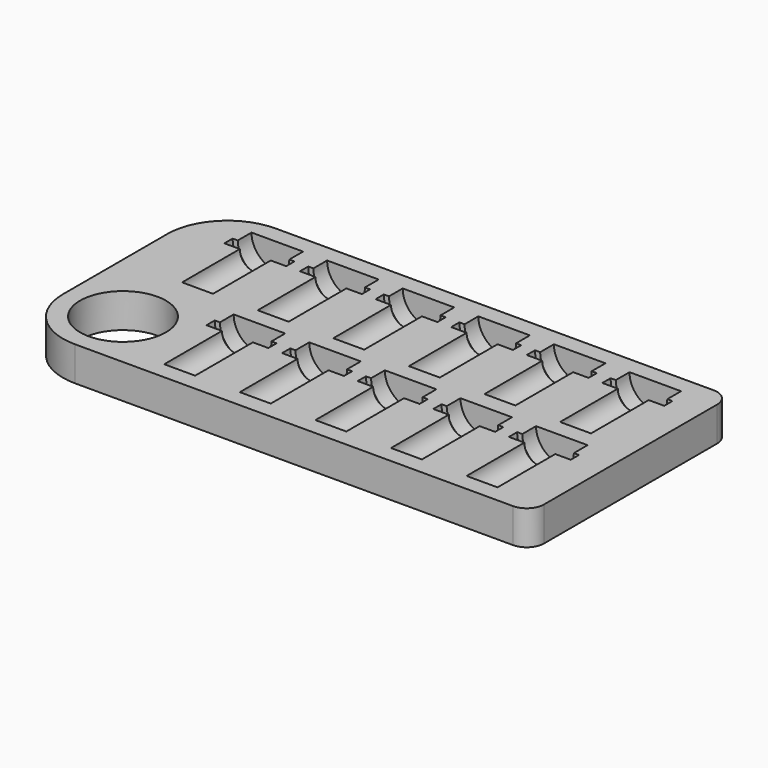
from build123d import *

# Parameters (mm, degrees)
F0_R         = 12.5
F1_DEPTH     = 10
F9_TEXT_SIZE = 5.5555555556
F10_DEPTH    = 1


# Not quite as in the source:
# - Text() gives the source's letters only with a copy of the font that has no kerning and outlines rounded to 1/6400 em; it was checked with that copy


with BuildPart() as f1:
    # F0 (on Top) → F1 (new body)
    with BuildSketch(Plane.XY):
        with BuildLine():
            ThreePointArc((0, 17.5), (5.1256313292, 5.1256313292), (17.5, 0))
            Line((17.5, 0), (145, 0))
            ThreePointArc((145, 0), (148.5355339059, 1.4644660941), (150, 5))
            Line((150, 5), (150, 68))
            ThreePointArc((150, 68), (148.5355339059, 71.5355339059), (145, 73))
            Line((145, 73), (17.5, 73))
            ThreePointArc((17.5, 73), (5.1256313292, 67.8743686708), (0, 55.5))
            Line((0, 55.5), (0, 17.5))
        make_face()
        with Locations((17.5, 17.5)):
            Circle(F0_R, mode=Mode.SUBTRACT)
    extrude(amount=F1_DEPTH)

    # F2 (on face) → F3 (revolve, cut)
    with BuildSketch(Plane.XY.offset(10)):
        Polygon((22, 60), (22, 39), (26.5, 39), (26.5, 60), (31, 60), (31, 63), (29.5, 63), (29.5, 68), (22, 68), (22, 63), align=None)
    revolve(axis=Axis((22, 49.5, 10), (0, 1, 0)), mode=Mode.SUBTRACT)

    # F2 (on face) → F4 (revolve, cut)
    with BuildSketch(Plane.XY.offset(10)):
        Polygon((44, 26), (44, 5), (48.5, 5), (48.5, 26), (53, 26), (53, 29), (51.5, 29), (51.5, 34), (44, 34), (44, 29), align=None)
        Polygon((44, 60), (44, 39), (48.5, 39), (48.5, 60), (53, 60), (53, 63), (51.5, 63), (51.5, 68), (44, 68), (44, 63), align=None)
    revolve(axis=Axis((44, 49.5, 10), (0, 1, 0)), mode=Mode.SUBTRACT)

    # F2 (on face) → F5 (revolve, cut)
    with BuildSketch(Plane.XY.offset(10)):
        Polygon((66, 26), (66, 5), (70.5, 5), (70.5, 26), (75, 26), (75, 29), (73.5, 29), (73.5, 34), (66, 34), (66, 29), align=None)
        Polygon((66, 60), (66, 39), (70.5, 39), (70.5, 60), (75, 60), (75, 63), (73.5, 63), (73.5, 68), (66, 68), (66, 63), align=None)
    revolve(axis=Axis((66, 49.5, 10), (0, 1, 0)), mode=Mode.SUBTRACT)

    # F2 (on face) → F6 (revolve, cut)
    with BuildSketch(Plane.XY.offset(10)):
        Polygon((88, 26), (88, 5), (92.5, 5), (92.5, 26), (97, 26), (97, 29), (95.5, 29), (95.5, 34), (88, 34), (88, 29), align=None)
        Polygon((88, 60), (88, 39), (92.5, 39), (92.5, 60), (97, 60), (97, 63), (95.5, 63), (95.5, 68), (88, 68), (88, 63), align=None)
    revolve(axis=Axis((88, 49.5, 10), (0, 1, 0)), mode=Mode.SUBTRACT)

    # F2 (on face) → F7 (revolve, cut)
    with BuildSketch(Plane.XY.offset(10)):
        Polygon((110, 26), (110, 5), (114.5, 5), (114.5, 26), (119, 26), (119, 29), (117.5, 29), (117.5, 34), (110, 34), (110, 29), align=None)
        Polygon((110, 60), (110, 39), (114.5, 39), (114.5, 60), (119, 60), (119, 63), (117.5, 63), (117.5, 68), (110, 68), (110, 63), align=None)
    revolve(axis=Axis((110, 49.5, 10), (0, 1, 0)), mode=Mode.SUBTRACT)

    # F2 (on face) → F8 (revolve, cut)
    with BuildSketch(Plane.XY.offset(10)):
        Polygon((132, 26), (132, 5), (136.5, 5), (136.5, 26), (141, 26), (141, 29), (139.5, 29), (139.5, 34), (132, 34), (132, 29), align=None)
        Polygon((132, 60), (132, 39), (136.5, 39), (136.5, 60), (141, 60), (141, 63), (139.5, 63), (139.5, 68), (132, 68), (132, 63), align=None)
    revolve(axis=Axis((132, 49.5, 10), (0, 1, 0)), mode=Mode.SUBTRACT)

    # F9 (on face) → F10 (cut)
    with BuildSketch(Plane(origin=(0, 0, 0), x_dir=(1, 0, 0), z_dir=(0, 0, -1))):
        with Locations((30, -9)):
            Text('791', F9_TEXT_SIZE, font='Open Sans', text_align=(TextAlign.LEFT, TextAlign.BOTTOM))
    extrude(amount=-F10_DEPTH, mode=Mode.SUBTRACT)


solid = f1.part
